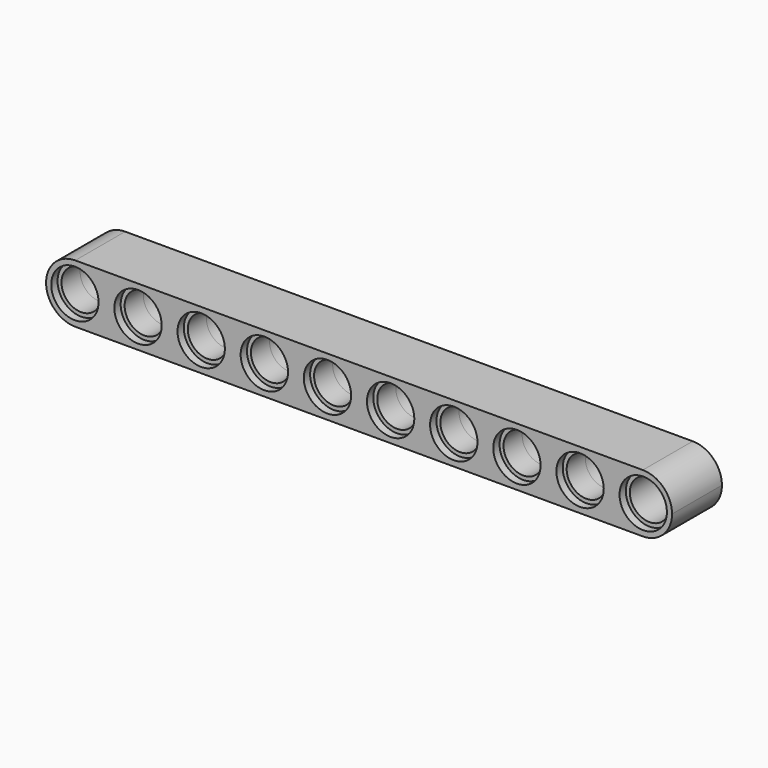
from build123d import *

# Parameters (mm, degrees)
F0_W     = 79.3
F0_H     = 7.4
F0_R     = 3
F1_DEPTH = 3.95
F0_R_2   = 2.499
F2_DEPTH = 2.95
F3_R     = 3.69999


# Not quite as in the source:
# - a fillet or chamfer is up to 0.001 mm smaller than in the source, because OpenCascade refuses the exact size


with BuildPart() as f1:
    # F0 (on Front) → F1 (new body, symmetric)
    with BuildSketch(Plane.XZ):
        with Locations((-4, 0)):
            Rectangle(F0_W, F0_H)
        with Locations((-40, 0)):
            Circle(F0_R, mode=Mode.SUBTRACT)
        with Locations((-32, 0)):
            Circle(F0_R, mode=Mode.SUBTRACT)
        with Locations((-24, 0)):
            Circle(F0_R, mode=Mode.SUBTRACT)
        with Locations((-16, 0)):
            Circle(F0_R, mode=Mode.SUBTRACT)
        with Locations((-8, 0)):
            Circle(F0_R, mode=Mode.SUBTRACT)
        Circle(F0_R, mode=Mode.SUBTRACT)
        with Locations((8, 0)):
            Circle(F0_R, mode=Mode.SUBTRACT)
        with Locations((16, 0)):
            Circle(F0_R, mode=Mode.SUBTRACT)
        with Locations((24, 0)):
            Circle(F0_R, mode=Mode.SUBTRACT)
        with Locations((32, 0)):
            Circle(F0_R, mode=Mode.SUBTRACT)
    extrude(amount=F1_DEPTH, both=True)

    # F0 (on Front) → F2 (join, symmetric)
    with BuildSketch(Plane.XZ):
        with Locations((-40, 0)):
            Circle(F0_R)
        with Locations((-40, 0)):
            Circle(F0_R_2, mode=Mode.SUBTRACT)
        with Locations((-32, 0)):
            Circle(F0_R)
        with Locations((-32, 0)):
            Circle(F0_R_2, mode=Mode.SUBTRACT)
        with Locations((-24, 0)):
            Circle(F0_R)
        with Locations((-24, 0)):
            Circle(F0_R_2, mode=Mode.SUBTRACT)
        with Locations((-16, 0)):
            Circle(F0_R)
        with Locations((-16, 0)):
            Circle(F0_R_2, mode=Mode.SUBTRACT)
        with Locations((-8, 0)):
            Circle(F0_R)
        with Locations((-8, 0)):
            Circle(F0_R_2, mode=Mode.SUBTRACT)
        Circle(F0_R)
        Circle(F0_R_2, mode=Mode.SUBTRACT)
        with Locations((8, 0)):
            Circle(F0_R)
        with Locations((8, 0)):
            Circle(F0_R_2, mode=Mode.SUBTRACT)
        with Locations((16, 0)):
            Circle(F0_R)
        with Locations((16, 0)):
            Circle(F0_R_2, mode=Mode.SUBTRACT)
        with Locations((24, 0)):
            Circle(F0_R)
        with Locations((24, 0)):
            Circle(F0_R_2, mode=Mode.SUBTRACT)
        with Locations((32, 0)):
            Circle(F0_R)
        with Locations((32, 0)):
            Circle(F0_R_2, mode=Mode.SUBTRACT)
    extrude(amount=F2_DEPTH, both=True)

    # F3 (radius 3.7 in the source; OpenCascade refuses exactly that, so slightly less here)
    f3_edges = [f1.edges().sort_by_distance(p)[0] for p in [
        (-43.65, 0, 3.7),
        (35.65, 0, 3.7),
        (35.65, 0, -3.7),
        (-43.65, 0, -3.7),
    ]]
    fillet(f3_edges, radius=F3_R)


solid = f1.part
